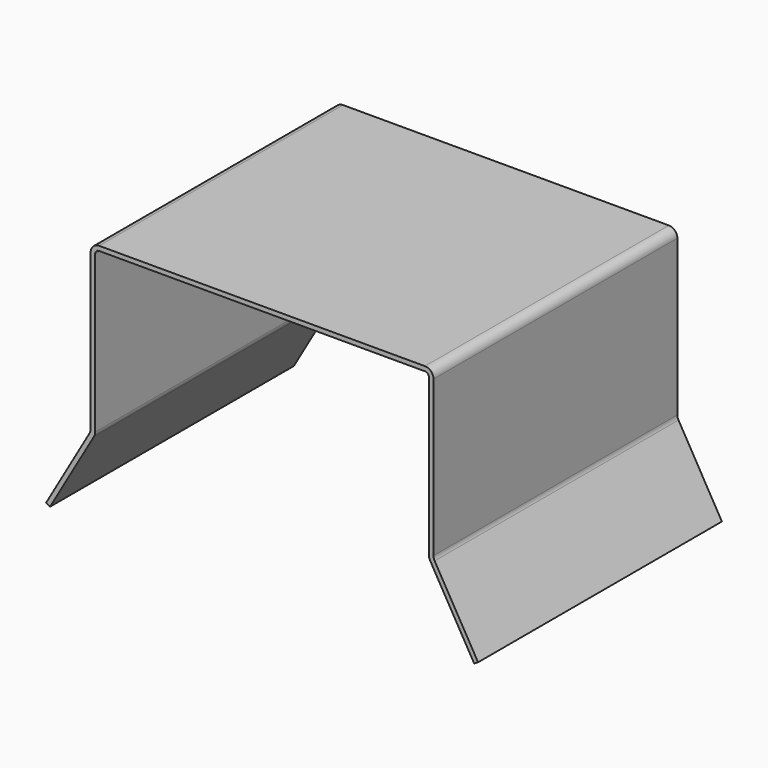
from build123d import *

# Parameters (mm, degrees)
F1_DEPTH = 177.8
F2_R     = 5


with BuildPart() as f1:
    # F0 (on Front) → F1 (new body)
    with BuildSketch(Plane.XZ):
        with BuildLine():
            Line((195, 0), (5, 0))
            ThreePointArc((5, 0), (1.4644660941, -1.4644660941), (0, -5))
            Line((0, -5), (0, -97))
            Line((0, -97), (-25.9807621135, -142))
            Line((-25.9807621135, -142), (-23.6857947935, -143.325))
            Line((-23.6857947935, -143.325), (2.65, -97.7100653599))
            Line((2.65, -97.7100653599), (2.65, -5))
            ThreePointArc((2.65, -5), (3.3382990642, -3.3382990642), (5, -2.65))
            Line((5, -2.65), (195, -2.65))
            ThreePointArc((195, -2.65), (196.6617009358, -3.3382990642), (197.35, -5))
            Line((197.35, -5), (197.35, -97.7100653599))
            Line((197.35, -97.7100653599), (223.6857947935, -143.325))
            Line((223.6857947935, -143.325), (225.9807621135, -142))
            Line((225.9807621135, -142), (200, -97))
            Line((200, -97), (200, -5))
            ThreePointArc((200, -5), (198.5355339059, -1.4644660941), (195, 0))
        make_face()
    extrude(amount=F1_DEPTH)

    # F2
    f2_edges = [f1.edges().sort_by_distance(p)[0] for p in [
        (200, -88.9, -97),
        (197.35, -88.9, -97.710065),
        (2.65, -88.9, -97.710065),
        (0, -88.9, -97),
    ]]
    fillet(f2_edges, radius=F2_R)


solid = f1.part
